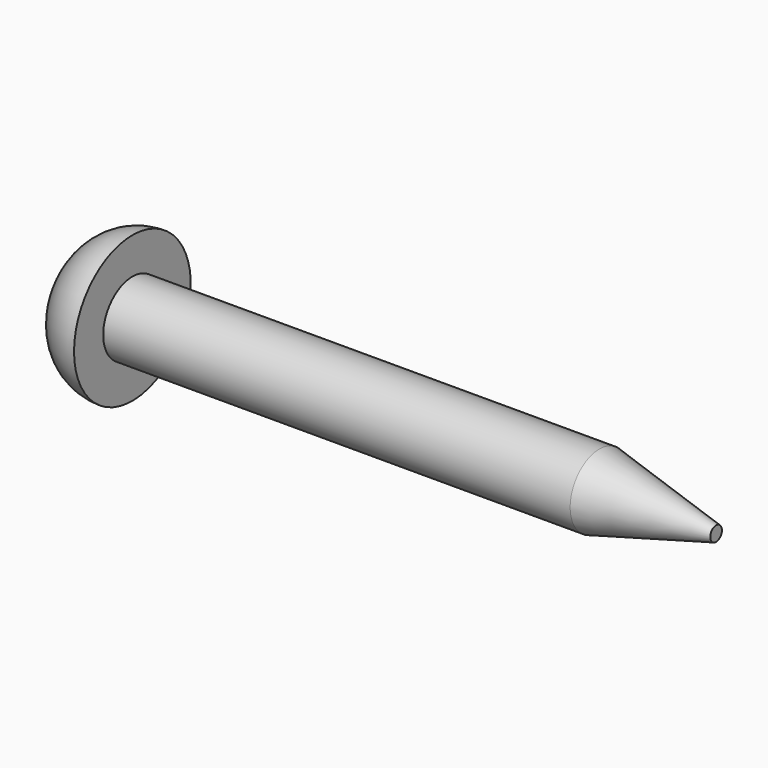
from build123d import *

# Parameters (mm, degrees)
F0_R     = 1.5875
F1_DEPTH = 25.4
F2_R     = 3.175
F2_R_2   = 1.5875
F3_DEPTH = 2.54
F4_R     = 2.53999
F5_SIZE2 = 5.08
F5_SIZE  = 1.27


# Not quite as in the source:
# - a fillet or chamfer is up to 0.001 mm smaller than in the source, because OpenCascade refuses the exact size


with BuildPart() as f1:
    # F0 (on Right) → F1 (new body)
    with BuildSketch(Plane.YZ):
        Circle(F0_R)
    extrude(amount=-F1_DEPTH)

    # F2 (on face) → F3 (join)
    with BuildSketch(Plane(origin=(-25.4, 0, 0), x_dir=(0, -1, 0), z_dir=(-1, 0, 0))):
        Circle(F2_R)
        Circle(F2_R_2, mode=Mode.SUBTRACT)
        Circle(F2_R_2)
    extrude(amount=F3_DEPTH)

    # F4 (radius 2.54 in the source; OpenCascade refuses exactly that, so slightly less here)
    f4_edges = [f1.edges().sort_by_distance(p)[0] for p in [
        (-27.94, 3.175, 0),
    ]]
    fillet(f4_edges, radius=F4_R)

    # F5
    f5_edges = [f1.edges().sort_by_distance(p)[0] for p in [
        (0, -1.5875, 0),
    ]]
    f5_side = f1.faces().sort_by_distance((0, 0, 0))[0]
    chamfer(f5_edges, length=F5_SIZE, length2=F5_SIZE2, reference=f5_side)


solid = f1.part
